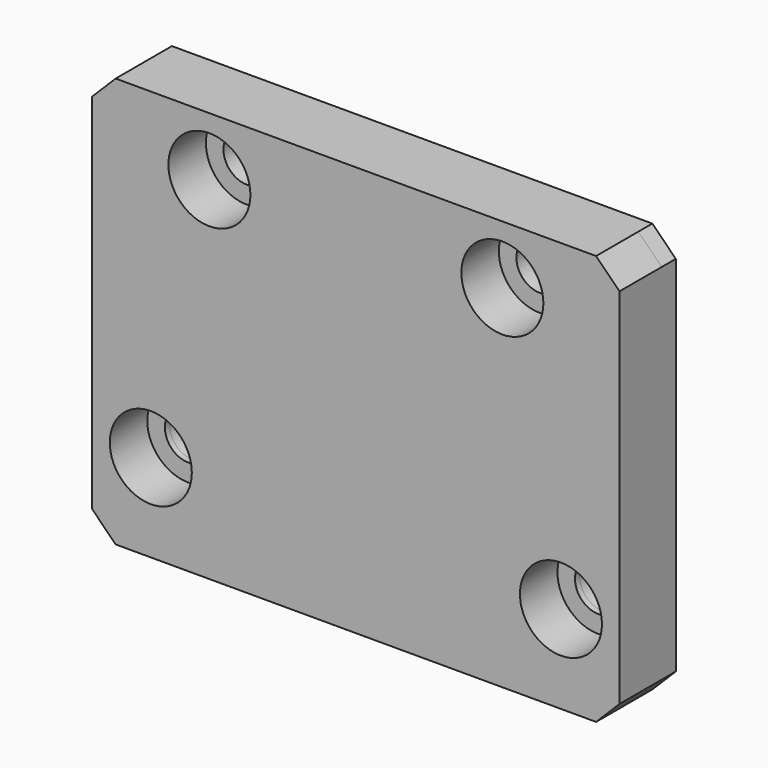
from build123d import *

# Parameters (mm, degrees)
F0_W      = 45
F0_H      = 35
F1_DEPTH  = 4.5
F2_W      = 15
F2_H      = 1.5
F3_DEPTH  = 35.001
F4_R      = 1.75
F5_DEPTH  = 3.5
F6_R      = 2
F7_DEPTH  = 4.501
F8_W      = 10
F8_H      = 10
F9_DEPTH  = 3
F10_SIZE  = 2
F11_W     = 48.3506806195
F11_H     = 3
F12_DEPTH = 35.001
F13_W     = 45
F13_H     = 35
F14_DEPTH = 4.5
F15_SIZE  = 1.99999
F16_R     = 2
F17_DEPTH = 6.001
F18_R     = 3.5
F19_DEPTH = 4
F20_R     = 3.5
F21_DEPTH = 4
F22_R     = 2
F23_DEPTH = 6.001


# Not quite as in the source:
# - a fillet or chamfer is up to 0.001 mm smaller than in the source, because OpenCascade refuses the exact size


with BuildPart() as f1:
    # F0 (on Front) → F1 (new body)
    with BuildSketch(Plane.XZ):
        with Locations((0, 2.5)):
            Rectangle(F0_W, F0_H)
    extrude(amount=F1_DEPTH)

    # F2 (on face) → F3 (cut, through all)
    with BuildSketch(Plane.XY.offset(20)):
        with Locations((-2.5, -2.25)):
            Rectangle(F2_W, F2_H)
    extrude(amount=-F3_DEPTH, mode=Mode.SUBTRACT)

    # F4 (on face) → F5 (cut)
    with BuildSketch(Plane.XZ.offset(4.5)):
        with Locations((17.5, -7.5)):
            Circle(F4_R)
        with Locations((-17.5, -7.5)):
            Circle(F4_R)
    extrude(amount=-F5_DEPTH, mode=Mode.SUBTRACT)

    # F6 (on face) → F7 (cut, through all)
    with BuildSketch(Plane.XZ.offset(4.5)):
        with Locations((17.5, -7.5)):
            Circle(F6_R)
        with Locations((-17.5, -7.5)):
            Circle(F6_R)
    extrude(amount=-F7_DEPTH, mode=Mode.SUBTRACT)

    # F8 (on face) → F9 (cut)
    with BuildSketch(Plane(origin=(0, 0, 0), x_dir=(-1, 0, 0), z_dir=(0, 1, 0))):
        with Locations((5, 10)):
            Rectangle(F8_W, F8_H)
    extrude(amount=-F9_DEPTH, mode=Mode.SUBTRACT)

    # F10
    f10_edges = [f1.edges().sort_by_distance(p)[0] for p in [
        (-22.5, -2.25, 20),
        (22.5, -2.25, 20),
        (22.5, -2.25, -15),
        (-22.5, -2.25, -15),
    ]]
    chamfer(f10_edges, length=F10_SIZE)

    # F11 (on face) → F12 (cut, through all)
    with BuildSketch(Plane(origin=(0, 0, -15), x_dir=(1, 0, 0), z_dir=(0, 0, -1))):
        with Locations((0.253405422, 1.5)):
            Rectangle(F11_W, F11_H)
    extrude(amount=-F12_DEPTH, mode=Mode.SUBTRACT)

    # F13 (on face) → F14 (join)
    with BuildSketch(Plane.XZ.offset(4.5)):
        with Locations((0, 2.5)):
            Rectangle(F13_W, F13_H)
    extrude(amount=F14_DEPTH)

    # F15 (size 2 in the source; OpenCascade refuses exactly that, so slightly less here)
    f15_edges = [f1.edges().sort_by_distance(p)[0] for p in [
        (-22.5, -6.75, -15),
        (22.5, -6.75, -15),
        (22.5, -6.75, 20),
        (-22.5, -6.75, 20),
    ]]
    chamfer(f15_edges, length=F15_SIZE)

    # F16 (on face) → F17 (cut, through all)
    with BuildSketch(Plane(origin=(0, -3, 0), x_dir=(-1, 0, 0), z_dir=(0, 1, 0))):
        with Locations((17.5, -7.5)):
            Circle(F16_R)
        with Locations((-17.5, -7.5)):
            Circle(F16_R)
    extrude(amount=-F17_DEPTH, mode=Mode.SUBTRACT)

    # F18 (on face) → F19 (cut)
    with BuildSketch(Plane.XZ.offset(9)):
        with Locations((-17.5, -7.5)):
            Circle(F18_R)
        with Locations((17.5, -7.5)):
            Circle(F18_R)
    extrude(amount=-F19_DEPTH, mode=Mode.SUBTRACT)

    # F20 (on face) → F21 (cut)
    with BuildSketch(Plane.XZ.offset(9)):
        with Locations((-12.5, 15)):
            Circle(F20_R)
        with Locations((12.5, 15)):
            Circle(F20_R)
    extrude(amount=-F21_DEPTH, mode=Mode.SUBTRACT)

    # F22 (on face) → F23 (cut, through all)
    with BuildSketch(Plane.XZ.offset(9)):
        with Locations((-12.5, 15)):
            Circle(F22_R)
        with Locations((12.5, 15)):
            Circle(F22_R)
    extrude(amount=-F23_DEPTH, mode=Mode.SUBTRACT)


solid = f1.part
